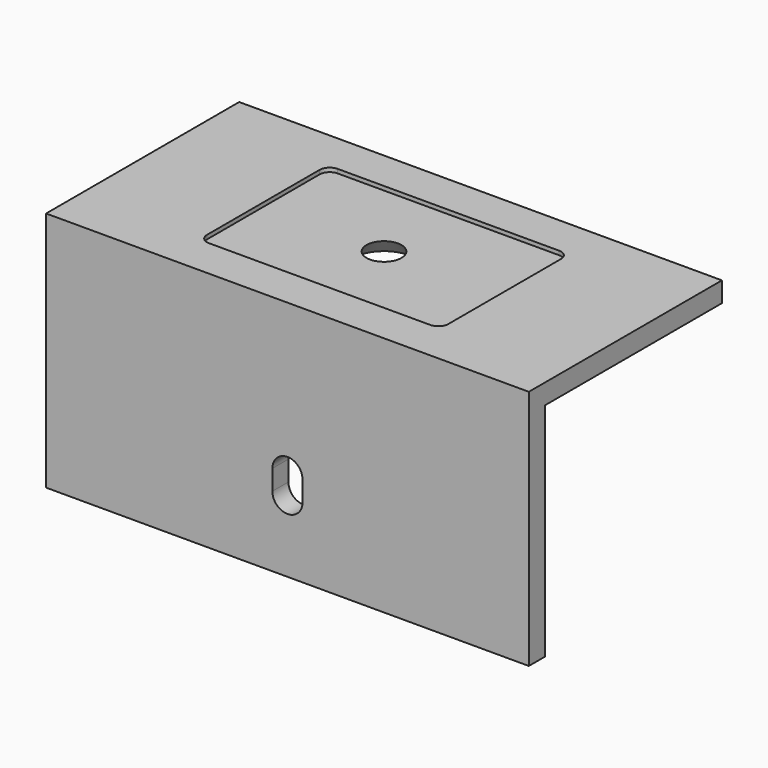
from build123d import *

# Parameters (mm, degrees)
F1_DEPTH       = 152.4
F3_D           = 9.525
F3_CSINK_D     = 19.8628
F3_CSINK_ANGLE = 82
F4_R           = 4.7625
F5_DEPTH       = 1.27
F7_DEPTH       = 76.201


# Not quite as in the source:
# - a length typed as a fraction of an inch, garbled in the dataset ("3 / 203.2 mm" for 3/8 in), is restored
# - a feature names something its author has since deleted; it is built from what else it names


with BuildPart() as f1:
    # F0 (on Right) → F1 (new body)
    with BuildSketch(Plane.YZ):
        Polygon((76.2, -6.35), (76.2, 0), (0, 0), (0, -76.2), (6.35, -76.2), (6.35, -6.35), align=None)
    extrude(amount=F1_DEPTH)

    # F3 (through all)
    with Locations(Plane(origin=(0, 0, -6.35), x_dir=(1, 0, 0), z_dir=(0, 0, -1))):
        with Locations((76.2, -38.1)):
            CounterSinkHole(F3_D / 2, F3_CSINK_D / 2, counter_sink_angle=F3_CSINK_ANGLE)

    # F4 (on face) → F5 (cut)
    with BuildSketch(Plane.XY):
        with BuildLine():
            Line((111.125, 63.5), (41.275, 63.5))
            ThreePointArc((41.275, 63.5), (39.0299359697, 62.5700640303), (38.1, 60.325))
            Line((38.1, 60.325), (38.1, 15.875))
            ThreePointArc((38.1, 15.875), (39.0299359697, 13.6299359697), (41.275, 12.7))
            Line((41.275, 12.7), (111.125, 12.7))
            ThreePointArc((111.125, 12.7), (113.3700640303, 13.6299359697), (114.3, 15.875))
            Line((114.3, 15.875), (114.3, 60.325))
            ThreePointArc((114.3, 60.325), (113.3700640303, 62.5700640303), (111.125, 63.5))
        make_face()
        with Locations((76.2, 38.1)):
            Circle(F4_R, mode=Mode.SUBTRACT)
    extrude(amount=-F5_DEPTH, mode=Mode.SUBTRACT)

    # F6 (on face) → F7 (cut, through all)
    with BuildSketch(Plane.XZ):
        with BuildLine():
            Line((71.4375, -47.625), (71.4375, -53.975))
            ThreePointArc((71.4375, -53.975), (76.2, -58.7375), (80.9625, -53.975))
            Line((80.9625, -53.975), (80.9625, -47.625))
            ThreePointArc((80.9625, -47.625), (76.2, -42.8625), (71.4375, -47.625))
        make_face()
    extrude(amount=-F7_DEPTH, mode=Mode.SUBTRACT)


solid = f1.part
